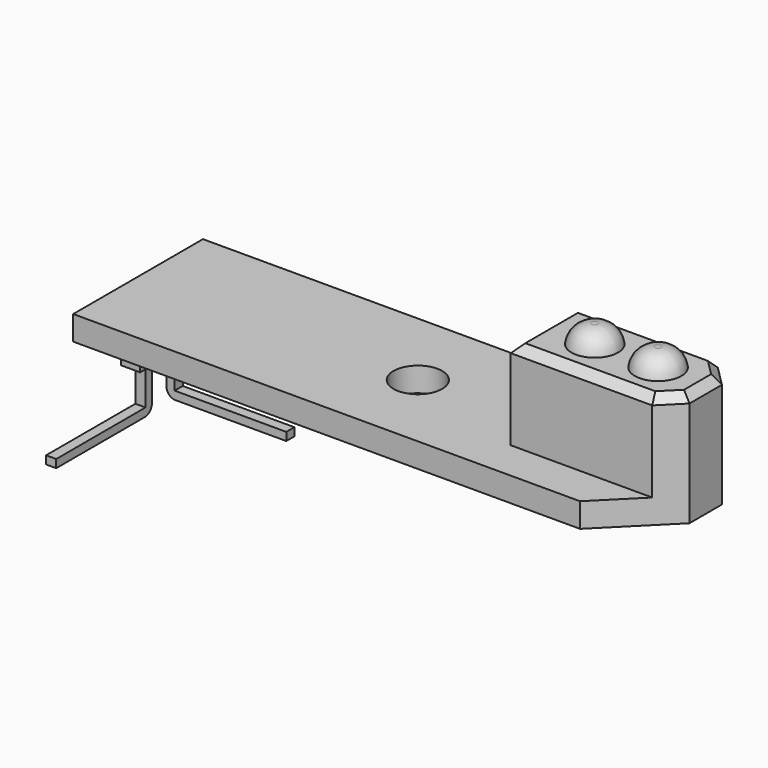
from build123d import *

# Parameters (mm, degrees)
F1_DEPTH  = 1.524
F3_DEPTH  = 5.588
F4_R      = 1.4605
F5_DEPTH  = 1.143
F7_SIZE   = 0.508
F9_DEPTH  = 0.3175
F11_ANGLE = 90
F13_ANGLE = 180
F15_W     = 1.2032650411
F15_H     = 6.585133262
F15_W_2   = 0.635
F15_H_2   = 0.508
F16_DEPTH = 1.524
F17_R     = 1.524
F18_DEPTH = 25.4


# Not quite as in the source:
# - a fillet or chamfer that OpenCascade refuses, or shapes differently, is made with other operations: its cross-section is extruded or revolved along the edge and cut away or added


with BuildPart() as f1:
    # F0 (on Top) → F1 (new body)
    with BuildSketch(Plane.XY):
        Polygon((-17.78, -5.08), (13.97, -5.08), (16.4832153797, -2.5667846203), (7.62, -2.5667846203), (7.62, 2.5667846203), (16.4832153797, 2.5667846203), (13.97, 5.08), (-17.78, 5.08), align=None)
        Polygon((7.62, -2.5667846203), (16.4832153797, -2.5667846203), (17.78, -1.27), (17.78, 1.27), (16.4832153797, 2.5667846203), (7.62, 2.5667846203), align=None)
    extrude(amount=-F1_DEPTH)

    # F2 (on face) → F3 (join)
    with BuildSketch(Plane.XY):
        Polygon((16.4832153797, -2.5667846203), (17.78, -1.27), (17.78, 1.27), (16.4832153797, 2.5667846203), (7.62, 2.5667846203), (7.62, -2.5667846203), align=None)
    extrude(amount=F3_DEPTH)

    # F4 (on face) → F5 (join)
    with BuildSketch(Plane.XY.offset(5.588)):
        with Locations((10.829353705, 0)):
            Circle(F4_R)
        with Locations((14.7973923013, 0)):
            Circle(F4_R)
    extrude(amount=F5_DEPTH)

    # F6: fillet of radius 1.27 on 2 edges, made by hand

    # F6_s1 → F6_t2 (revolve, cut)
    with BuildSketch(Plane.XZ):
        with BuildLine():
            ThreePointArc((12.289853705, 5.588), (11.8781615594, 6.4028572079), (11.0262196599, 6.731))
            Line((11.0262196599, 6.731), (12.289853705, 6.731))
            Line((12.289853705, 6.731), (12.289853705, 5.588))
        make_face()
    revolve(axis=Axis((10.829353705, 0, 6.731), (0, 0, 1)), mode=Mode.SUBTRACT)

    # F6_s3 → F6_t4 (revolve, cut)
    with BuildSketch(Plane.XZ):
        with BuildLine():
            ThreePointArc((16.2578923013, 5.588), (15.8462001556, 6.4028572079), (14.9942582561, 6.731))
            Line((14.9942582561, 6.731), (16.2578923013, 6.731))
            Line((16.2578923013, 6.731), (16.2578923013, 5.588))
        make_face()
    revolve(axis=Axis((14.7973923013, 0, 6.731), (0, 0, 1)), mode=Mode.SUBTRACT)

    # F7
    f7_edges = [f1.edges().sort_by_distance(p)[0] for p in [
        (12.051608, -2.566785, 5.588),
        (12.051608, 2.566785, 5.588),
        (7.62, 0, 5.588),
        (17.78, 0, 5.588),
        (17.131608, -1.918392, 5.588),
        (17.131608, 1.918392, 5.588),
    ]]
    chamfer(f7_edges, length=F7_SIZE)

    # F12: F10_1 across plane


with BuildPart() as f9:
    # F8 (on Front) → F9 (new body, symmetric)
    with BuildSketch(Plane.XZ):
        with BuildLine():
            Line((-22.86, -5.334), (-22.86, -5.842))
            Line((-22.86, -5.842), (-15.9157037269, -5.842))
            ThreePointArc((-15.9157037269, -5.842), (-15.5230394847, -5.6793531454), (-15.3603926301, -5.2866889032))
            Line((-15.3603926301, -5.2866889032), (-15.3603926301, -1.1672781548))
            Line((-15.3603926301, -1.1672781548), (-15.8683926301, -1.1672781548))
            Line((-15.8683926301, -1.1672781548), (-15.8683926301, -5.334))
            Line((-15.8683926301, -5.334), (-22.86, -5.334))
        make_face()
    extrude(amount=F9_DEPTH, both=True)


with BuildPart() as f10_1:
    # F10: copy of F9
    add(f9.part.moved(Location((0, -2.92, 0))))


with BuildPart() as f10_1_1:
    # F11: moved
    add(f10_1.part.rotate(Axis((-15.8683926301, -2.6025, -3.2506390774), (0, 0, 1)), F11_ANGLE))


with BuildPart() as f1_1:
    add(f1.part)
    add(f10_1_1.part.mirror(Plane.XZ))



with BuildPart() as f9_1:
    # F13: moved
    add(f9.part.rotate(Axis((-15.8683926301, 0.3175, -3.2506390774), (0, 0, 1)), F13_ANGLE))


with BuildPart() as f9_2:
    # F14: moved
    add(f9_1.part.moved(Location((0.635, -0.635, 0))))


with BuildPart() as f1_2:
    add(f1_1.part)

    add(f9_2.part)  # F16 merges F9

    add(f10_1_1.part)  # F16 merges F10_1
    # F15 (on face) → F16 (join)
    with BuildSketch(Plane(origin=(0, 0, -1.524), x_dir=(1, 0, 0), z_dir=(0, 0, -1))):
        with Locations((-15.6205464154, 0)):
            Rectangle(F15_W, F15_H)
        with Locations((-15.5508926301, -2.3485)):
            Rectangle(F15_W_2, F15_H_2, mode=Mode.SUBTRACT)
    extrude(amount=F16_DEPTH)

    # F17 (on face) → F18 (cut)
    with BuildSketch(Plane(origin=(0, 0, -1.524), x_dir=(1, 0, 0), z_dir=(0, 0, -1))):
        with Locations((-0.254, 0)):
            Circle(F17_R)
    extrude(amount=-F18_DEPTH, mode=Mode.SUBTRACT)


solid = f1_2.part
